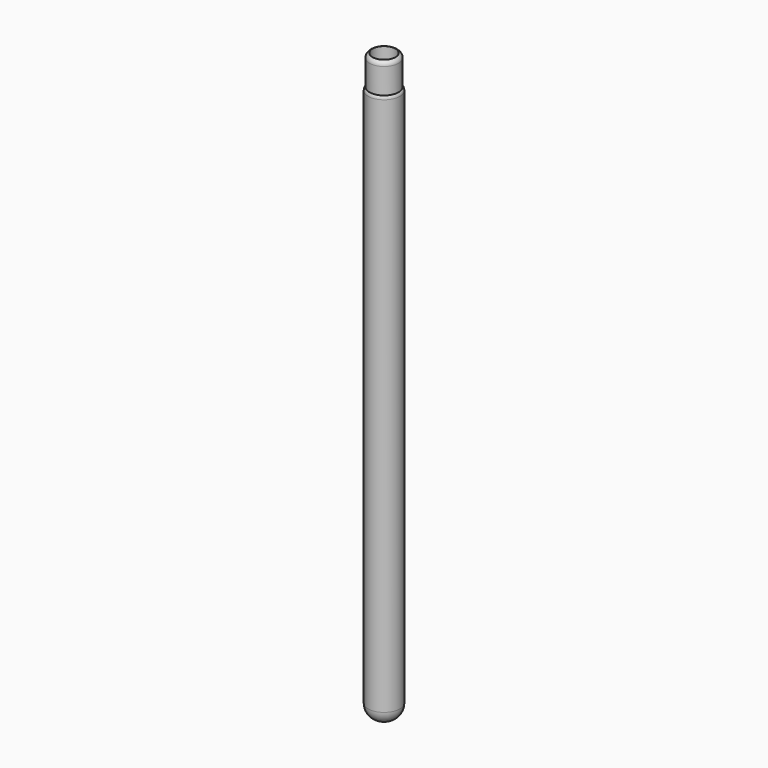
from build123d import *

# Parameters (mm, degrees)
F0_R     = 0.69
F0_R_2   = 0.635
F1_DEPTH = 24.2
F0_R_3   = 0.5
F2_DEPTH = 25.5
F3_DEPTH = 1
F4_R     = 0.6


# Not quite as in the source:
# - a fillet or chamfer that OpenCascade refuses, or shapes differently, is made with other operations: its cross-section is extruded or revolved along the edge and cut away or added


with BuildPart() as f1:
    # F0 (on Top) → F1 (new body)
    with BuildSketch(Plane.XY):
        Circle(F0_R)
        Circle(F0_R_2, mode=Mode.SUBTRACT)
    extrude(amount=F1_DEPTH)

    # F0 (on Top) → F2 (join)
    with BuildSketch(Plane.XY):
        Circle(F0_R_2)
        Circle(F0_R_3, mode=Mode.SUBTRACT)
    extrude(amount=F2_DEPTH)

    # F0 (on Top) → F3 (join)
    with BuildSketch(Plane.XY):
        Circle(F0_R)
        Circle(F0_R_2, mode=Mode.SUBTRACT)
        Circle(F0_R_2)
        Circle(F0_R_3, mode=Mode.SUBTRACT)
        Circle(F0_R_3)
    extrude(amount=F3_DEPTH)

    # F4
    f4_edges = [f1.edges().sort_by_distance(p)[0] for p in [
        (-0.69, 0, 0),
    ]]
    fillet(f4_edges, radius=F4_R)

    # F5: fillet of radius 0.2 on 2 edges, made by hand

    # F5_s1 → F5_t2 (revolve, cut)
    with BuildSketch(Plane.XZ):
        with BuildLine():
            ThreePointArc((0.69, 24.0622502269), (0.6757417562, 24.1364122117), (0.635, 24.2))
            Line((0.635, 24.2), (0.69, 24.2))
            Line((0.69, 24.2), (0.69, 24.0622502269))
        make_face()
    revolve(axis=Axis((0, 0, 24.2), (0, 0, 1)), mode=Mode.SUBTRACT)

    # F5_s3 → F5_t4 (revolve, cut)
    with BuildSketch(Plane.XZ):
        with BuildLine():
            ThreePointArc((0.635, 25.3108571968), (0.597788206, 25.4270466972), (0.5, 25.5))
            Line((0.5, 25.5), (0.635, 25.5))
            Line((0.635, 25.5), (0.635, 25.3108571968))
        make_face()
    revolve(axis=Axis((0, 0, 25.5), (0, 0, 1)), mode=Mode.SUBTRACT)


solid = f1.part
